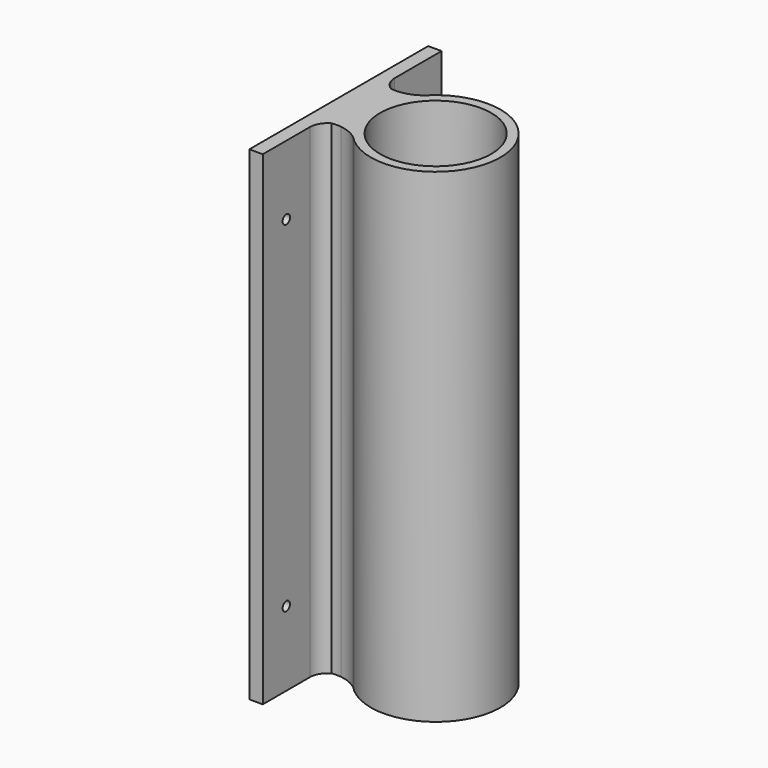
from build123d import *

# Parameters (mm, degrees)
F0_R        = 9.4742
F1_DEPTH    = 82.55
F2_R        = 9.4742
F3_DEPTH    = 2.286
F4_W        = 12.7000000767
F4_H        = 82.55
F4_W_2      = 12.7
F5_DEPTH    = 2.286
F6_T1_DEPTH = 82.55
F7_R        = 0.7874
F8_DEPTH    = 13.208


# Not quite as in the source:
# - a fillet or chamfer that OpenCascade refuses, or shapes differently, is made with other operations: its cross-section is extruded or revolved along the edge and cut away or added
# - a pattern or mirror of a feature is missing from the dataset's text; its kind, count and spacing are read off the source's solid


with BuildPart() as f1:
    # F0 (on Top) → F1 (new body)
    with BuildSketch(Plane.XY):
        with BuildLine():
            ThreePointArc((-11.049, -6.3499999233), (-9.4295157118, -6.785458523), (-7.9847846533, -7.6369899201))
            ThreePointArc((-7.9847846533, -7.6369899201), (-7.5622828297, -8.001877119), (-7.1741300574, -8.4031100742))
            ThreePointArc((-7.1741300574, -8.4031100742), (11.0467672464, 0.2221134929), (-7.5061119691, 8.1079395723))
            ThreePointArc((-7.5061119691, 8.1079395723), (-7.6290075774, 7.9871909027), (-7.755263928, 7.8699607628))
            ThreePointArc((-7.755263928, 7.8699607628), (-9.2865444962, 6.859503776), (-11.049, 6.35))
            ThreePointArc((-11.049, 6.35), (-11.84275, 6.2981423564), (-12.6365, 6.35))
            Line((-12.6365, 6.35), (-14.224, 6.35))
            Line((-14.224, 6.35), (-14.224, -6.3499999233))
            Line((-14.224, -6.3499999233), (-12.6365, -6.3499999233))
            ThreePointArc((-12.6365, -6.3499999233), (-11.84275, -6.2992439038), (-11.049, -6.3499999233))
        make_face()
        Circle(F0_R, mode=Mode.SUBTRACT)
    extrude(amount=F1_DEPTH)

    # F2 (on face) → F3 (join)
    with BuildSketch(Plane(origin=(0, 0, 0), x_dir=(1, 0, 0), z_dir=(0, 0, -1))):
        Circle(F2_R)
    extrude(amount=-F3_DEPTH)

    # F4 (on face) → F5 (join)
    with BuildSketch(Plane(origin=(-14.224, 0, 0), x_dir=(0, -1, 0), z_dir=(-1, 0, 0))):
        Polygon((6.3499999233, 82.55), (0, 82.55), (-6.35, 82.55), (-6.35, 0), (6.3499999233, 0), align=None)
        with Locations((12.6999999616, 41.275)):
            Rectangle(F4_W, F4_H)
        with Locations((-12.7, 41.275)):
            Rectangle(F4_W_2, F4_H)
    extrude(amount=F5_DEPTH)

    # F6: fillet of radius 3.048 on 2 edges, made by hand

    # F6_s2 → F6_t1 (join)
    with BuildSketch(Plane.XY):
        with BuildLine():
            ThreePointArc((-14.224, -9.0253024762), (-13.7972504649, -7.4698764896), (-12.6365, -6.3499999233))
            Line((-12.6365, -6.3499999233), (-14.224, -6.3499999233))
            Line((-14.224, -6.3499999233), (-14.224, -9.0253024762))
        make_face()
        with BuildLine():
            ThreePointArc((-14.224, 9.025302553), (-13.7972504649, 7.4698765663), (-12.6365, 6.35))
            Line((-12.6365, 6.35), (-14.224, 6.35))
            Line((-14.224, 6.35), (-14.224, 9.025302553))
        make_face()
    extrude(amount=F6_T1_DEPTH)

    # F7 (on face) → F8 (cut)
    with BuildSketch(Plane.YZ.offset(-14.224)):
        with Locations((-14.0376512381, 70.7353055477)):
            Circle(F7_R)
        with Locations((-14.0376512381, 12.7)):
            Circle(F7_R)
    f8 = extrude(amount=-F8_DEPTH, mode=Mode.SUBTRACT)

    # F8_copies: F8 across plane
    add(f8.mirror(Plane.ZX), mode=Mode.SUBTRACT)


solid = f1.part
